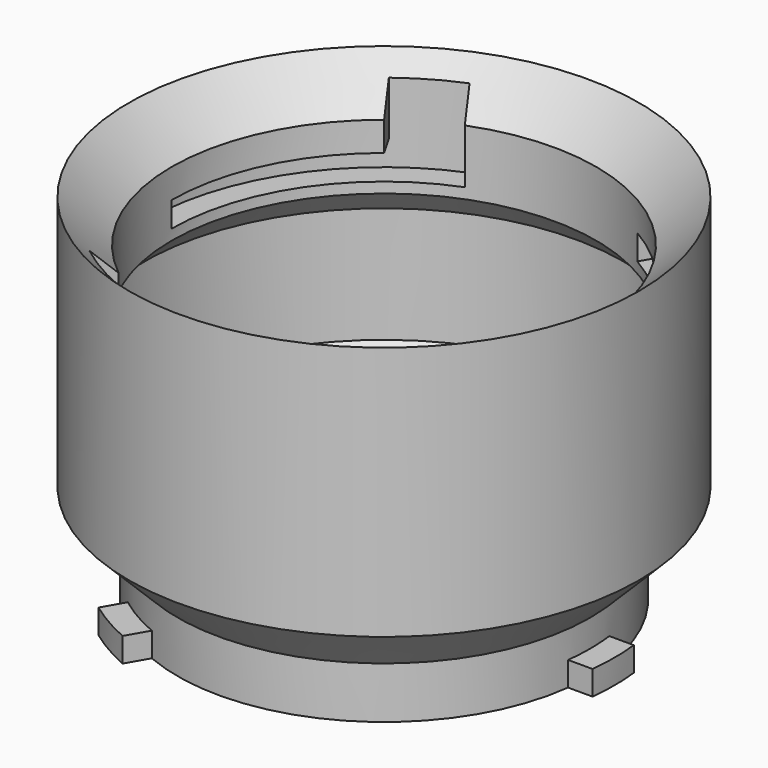
from build123d import *

# Parameters (mm, degrees)
F0_R             = 25.4
F1_DEPTH         = 6.35
F3_DEPTH         = 3
F4_R             = 22.4
F5_DEPTH         = 3.35
F6_R             = 31.4
F6_R_2           = 22.4
F7_DEPTH         = 31.75
F9_DEPTH         = 6.35
F10_R            = 26.15
F11_DEPTH        = 28
F12_W            = 10.4017283041
F12_H            = 3.1
F14_COPIES_COUNT = 3
F16_SIZE         = 5.99999
F17_R            = 31.4
F17_R_2          = 26.15
F18_DEPTH        = 6.35
F20_DEPTH        = 25


# Not quite as in the source:
# - a fillet or chamfer that OpenCascade refuses, or shapes differently, is made with other operations: its cross-section is extruded or revolved along the edge and cut away or added
# - a fillet or chamfer is up to 0.001 mm smaller than in the source, because OpenCascade refuses the exact size
# - a pattern or mirror of a feature is missing from the dataset's text; its kind, count and spacing are read off the source's solid


with BuildPart() as f1:
    # F0 (on Top) → F1 (new body)
    with BuildSketch(Plane.XY):
        Circle(F0_R)
    extrude(amount=-F1_DEPTH)

    # F2 (on face) → F3 (join)
    with BuildSketch(Plane(origin=(0, 0, -6.35), x_dir=(1, 0, 0), z_dir=(0, 0, -1))):
        with BuildLine():
            ThreePointArc((28.2219661788, -3.175), (28.4, 0), (28.2219661788, 3.175))
            Line((28.2219661788, 3.175), (22.4, 3.175))
            Line((22.4, 3.175), (22.4, -3.175))
            Line((22.4, -3.175), (28.2219661788, -3.175))
        make_face()
        with BuildLine():
            Line((-8.450369343, 20.9864690448), (-11.3613524324, 26.0284396556))
            ThreePointArc((-11.3613524324, 26.0284396556), (-14.2, 24.5951214675), (-16.8606137464, 22.8534396556))
            Line((-16.8606137464, 22.8534396556), (-13.949630657, 17.8114690448))
            Line((-13.949630657, 17.8114690448), (-8.450369343, 20.9864690448))
        make_face()
        with BuildLine():
            Line((-13.949630657, -17.8114690448), (-16.8606137464, -22.8534396556))
            ThreePointArc((-16.8606137464, -22.8534396556), (-14.2, -24.5951214675), (-11.3613524324, -26.0284396556))
            Line((-11.3613524324, -26.0284396556), (-8.450369343, -20.9864690448))
            Line((-8.450369343, -20.9864690448), (-13.949630657, -17.8114690448))
        make_face()
    extrude(amount=-F3_DEPTH)

    # F4 (on face) → F5 (cut, through all)
    with BuildSketch(Plane.XY):
        Circle(F4_R)
    extrude(amount=-F5_DEPTH, mode=Mode.SUBTRACT)

    # F6 (on face) → F7 (join)
    with BuildSketch(Plane.XY):
        Circle(F6_R)
        Circle(F6_R_2, mode=Mode.SUBTRACT)
    extrude(amount=F7_DEPTH)

    # F8 (on face) → F9 (cut)
    with BuildSketch(Plane.XY.offset(31.75)):
        with BuildLine():
            Line((17.4498241395, -3.925), (28.8845438773, -3.925))
            ThreePointArc((28.8845438773, -3.925), (29.15, 0), (28.8845438773, 3.925))
            Line((28.8845438773, 3.925), (17.4498241395, 3.925))
            Line((17.4498241395, 3.925), (17.4498241395, 0))
            Line((17.4498241395, 0), (17.4498241395, -3.925))
        make_face()
        with BuildLine():
            Line((-5.3257623599, 17.0744909964), (-11.0431222288, 26.9772487745))
            ThreePointArc((-11.0431222288, 26.9772487745), (-14.575, 25.2446405203), (-17.8414216485, 23.0522487745))
            Line((-17.8414216485, 23.0522487745), (-12.1240617796, 13.1494909964))
            Line((-12.1240617796, 13.1494909964), (-8.7249120697, 15.1119909964))
            Line((-8.7249120697, 15.1119909964), (-5.3257623599, 17.0744909964))
        make_face()
        with BuildLine():
            Line((-12.1240617796, -13.1494909964), (-17.8414216485, -23.0522487745))
            ThreePointArc((-17.8414216485, -23.0522487745), (-14.575, -25.2446405203), (-11.0431222288, -26.9772487745))
            Line((-11.0431222288, -26.9772487745), (-5.3257623599, -17.0744909964))
            Line((-5.3257623599, -17.0744909964), (-8.7249120697, -15.1119909964))
            Line((-8.7249120697, -15.1119909964), (-12.1240617796, -13.1494909964))
        make_face()
    extrude(amount=-F9_DEPTH, mode=Mode.SUBTRACT)

    # F10 (on face) → F11 (cut)
    with BuildSketch(Plane.XY.offset(31.75)):
        Circle(F10_R)
    extrude(amount=-F11_DEPTH, mode=Mode.SUBTRACT)

    # F14: sweep along a path in F13
    with BuildLine(Plane.XY.offset(31.75)) as f14_path:
        ThreePointArc((37.4274057464, 0), (32.4130841741, 18.7137028732), (18.7137028732, 32.4130841741))
    # F12 (on Front) → F14 (sweep, cut)
    with BuildSketch(Plane.XZ):
        with Locations((23.949135848, 26.95)):
            Rectangle(F12_W, F12_H)
    f14 = sweep(path=f14_path.line, mode=Mode.SUBTRACT)

    # F14_copies: F14 ×3 about axis
    f14_copies_axis = Axis((0, 0, 0), (0, 0, 1))
    for i in range(1, F14_COPIES_COUNT):
        add(f14.rotate(f14_copies_axis, i * 360 / F14_COPIES_COUNT), mode=Mode.SUBTRACT)

    # F16 (size 6 in the source; OpenCascade refuses exactly that, so slightly less here)
    f16_edges = [f1.edges().sort_by_distance(p)[0] for p in [
        (-31.4, 0, 0),
    ]]
    chamfer(f16_edges, length=F16_SIZE)

    # F17 (on face) → F18 (join)
    with BuildSketch(Plane.XY.offset(31.75)):
        Circle(F17_R)
        Circle(F17_R_2, mode=Mode.SUBTRACT)
    extrude(amount=F18_DEPTH)

    # F19: chamfer of 6 on 1 edges, made by hand

    # F19_s1 → F19_t2 (revolve, cut)
    with BuildSketch(Plane.XZ):
        Polygon((32.15, 38.1), (26.15, 32.1), (26.15, 38.1), align=None)
    revolve(axis=Axis((0, 0, 38.1), (0, 0, 1)), mode=Mode.SUBTRACT)

    # F8 (on face) → F20 (cut)
    with BuildSketch(Plane.XY.offset(31.75)):
        with BuildLine():
            Line((17.4498241395, -3.925), (28.8845438773, -3.925))
            ThreePointArc((28.8845438773, -3.925), (29.15, 0), (28.8845438773, 3.925))
            Line((28.8845438773, 3.925), (17.4498241395, 3.925))
            Line((17.4498241395, 3.925), (17.4498241395, 0))
            Line((17.4498241395, 0), (17.4498241395, -3.925))
        make_face()
        with BuildLine():
            Line((-5.3257623599, 17.0744909964), (-11.0431222288, 26.9772487745))
            ThreePointArc((-11.0431222288, 26.9772487745), (-14.575, 25.2446405203), (-17.8414216485, 23.0522487745))
            Line((-17.8414216485, 23.0522487745), (-12.1240617796, 13.1494909964))
            Line((-12.1240617796, 13.1494909964), (-8.7249120697, 15.1119909964))
            Line((-8.7249120697, 15.1119909964), (-5.3257623599, 17.0744909964))
        make_face()
        with BuildLine():
            Line((-12.1240617796, -13.1494909964), (-17.8414216485, -23.0522487745))
            ThreePointArc((-17.8414216485, -23.0522487745), (-14.575, -25.2446405203), (-11.0431222288, -26.9772487745))
            Line((-11.0431222288, -26.9772487745), (-5.3257623599, -17.0744909964))
            Line((-5.3257623599, -17.0744909964), (-8.7249120697, -15.1119909964))
            Line((-8.7249120697, -15.1119909964), (-12.1240617796, -13.1494909964))
        make_face()
    extrude(amount=F20_DEPTH, mode=Mode.SUBTRACT)

    # F21 (on Front) → F22 (revolve, cut)
    with BuildSketch(Plane.XZ):
        Polygon((0, 0), (0, -4.85), (23, -4.85), (23, 0), (29.5, 6.5), (29.5, 20.7537593978), (25.8537593978, 24.4), (0, 24.4), align=None)
    revolve(axis=Axis((0, 0, 37.5208705664), (0, 0, 1)), mode=Mode.SUBTRACT)


solid = f1.part
